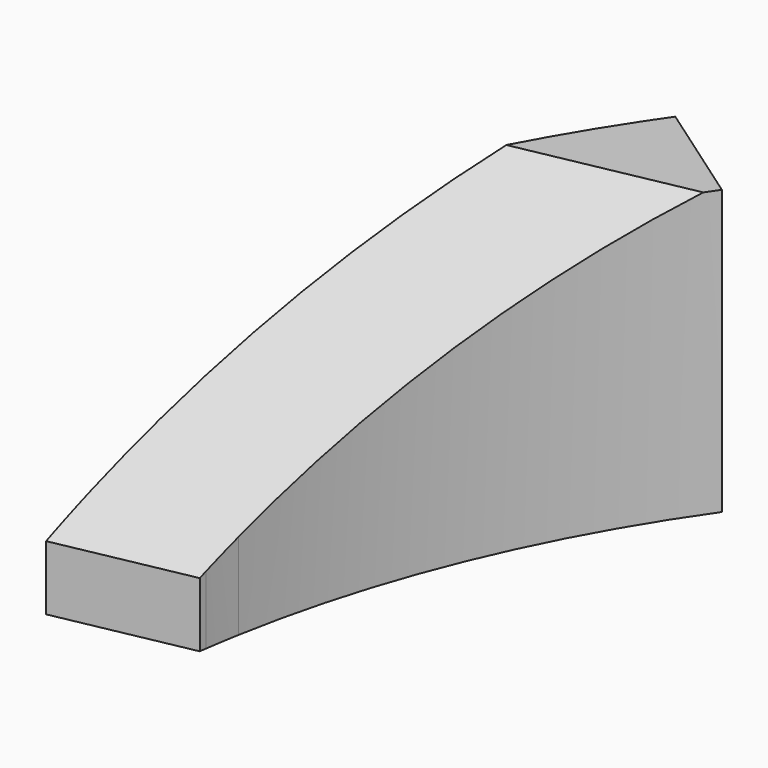
from build123d import *

# Parameters (mm, degrees)
F0_R        = 1.5
F1_DEPTH    = 22
F2_T1_DEPTH = 165.7438624109
F3_DEPTH    = 10


# Not quite as in the source:
# - a fillet or chamfer that OpenCascade refuses, or shapes differently, is made with other operations: its cross-section is extruded or revolved along the edge and cut away or added


with BuildPart() as f1:
    # F0 (on Top) → F1 (new body)
    with BuildSketch(Plane.XY):
        with BuildLine():
            ThreePointArc((-76.7321565298, 10.8823781538), (-76.533256864, 12.202892845), (-76.3116336523, 13.5197843663))
            Line((-76.3116336523, 13.5197843663), (-84.2766601783, 11.9523616575))
            Line((-84.2766601783, 11.9523616575), (-76.7321565298, 10.8823781538))
        make_face()
        with BuildLine():
            ThreePointArc((-76.3116336523, 13.5197843663), (-71.9683443093, 28.7542591172), (-64.6180706596, 42.7873222372))
            Line((-64.6180706596, 42.7873222372), (-72.9558862286, 48.3082670421))
            ThreePointArc((-72.9558862286, 48.3082670421), (-81.8018975861, 31.0596128649), (-86.633079953, 12.2865559801))
            Line((-86.633079953, 12.2865559801), (-84.2766601783, 11.9523616575))
            Line((-84.2766601783, 11.9523616575), (-76.3116336523, 13.5197843663))
        make_face()
        with Locations((-79.5430595227, 21.8895336125)):
            Circle(F0_R, mode=Mode.SUBTRACT)
        with Locations((-72.3838330612, 39.5832124944)):
            Circle(F0_R, mode=Mode.SUBTRACT)
        with BuildLine():
            ThreePointArc((-64.6180706596, 42.7873222372), (-64.076826103, 43.5936962939), (-63.5255193134, 44.3932246628))
            Line((-63.5255193134, 44.3932246628), (-71.7223605151, 50.1213826839))
            ThreePointArc((-71.7223605151, 50.1213826839), (-72.3448036647, 49.218689364), (-72.9558862286, 48.3082670421))
            Line((-72.9558862286, 48.3082670421), (-64.6180706596, 42.7873222372))
        make_face()
        with BuildLine():
            ThreePointArc((-76.8036989266, 10.365415148), (-76.7683628871, 10.6239568725), (-76.7321565298, 10.8823781538))
            Line((-76.7321565298, 10.8823781538), (-84.2766601783, 11.9523616575))
            Line((-84.2766601783, 11.9523616575), (-86.7454235032, 11.466538329))
            ThreePointArc((-86.7454235032, 11.466538329), (-86.9376476661, 9.9043131153), (-87.1017395415, 8.3388829496))
            Line((-87.1017395415, 8.3388829496), (-76.8036989266, 10.365415148))
        make_face()
        with BuildLine():
            Line((-86.7454235032, 11.466538329), (-84.2766601783, 11.9523616575))
            Line((-84.2766601783, 11.9523616575), (-86.633079953, 12.2865559801))
            ThreePointArc((-86.633079953, 12.2865559801), (-86.6902213195, 11.8766799899), (-86.7454235032, 11.466538329))
        make_face()
        with Locations((-72.3838330612, 39.5832124944)):
            Circle(F0_R)
        with Locations((-79.5430595227, 21.8895336125)):
            Circle(F0_R)
    extrude(amount=F1_DEPTH)

    # F2: chamfer of 17 x 30 on 1 edges, made by hand

    # F2_s2 → F2_t1 (cut)
    with BuildSketch(Plane(origin=(-158.4380449398, -31.1787272483, 0), x_dir=(0, 0, 1), z_dir=(0.9811820369, 0.1930849823, 0))):
        Polygon((5, -25), (22, -55), (22, -25), align=None)
    extrude(amount=F2_T1_DEPTH, mode=Mode.SUBTRACT)

    # F0 (on Top) → F3 (cut)
    with BuildSketch(Plane.XY):
        with Locations((-72.3838330612, 39.5832124944)):
            Circle(F0_R)
        with Locations((-79.5430595227, 21.8895336125)):
            Circle(F0_R)
    extrude(amount=F3_DEPTH, mode=Mode.SUBTRACT)


solid = f1.part
